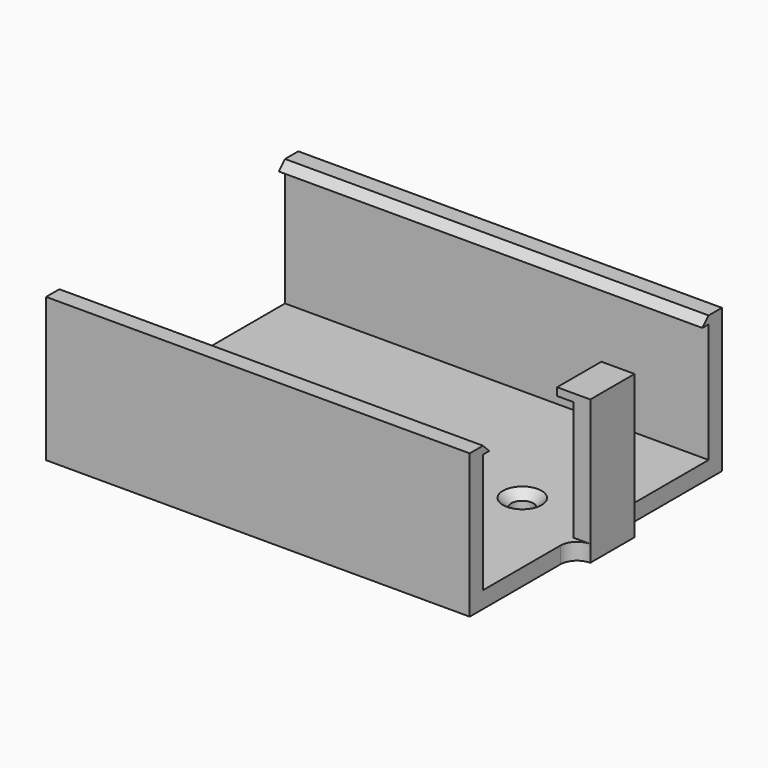
from build123d import *

# Parameters (mm, degrees)
F1_DEPTH        = 38.3
F2_W            = 76.6
F2_H            = 51
F3_DEPTH        = 19.6
F5_DEPTH        = 76.6
F7_DEPTH        = 3
F8_W            = 10
F8_H            = 21.6
F9_DEPTH        = 3
F10_R           = 2.99999
F12_D           = 4
F12_CSINK_D     = 7
F12_CSINK_ANGLE = 90


# Not quite as in the source:
# - a fillet or chamfer is up to 0.001 mm smaller than in the source, because OpenCascade refuses the exact size


with BuildPart() as f1:
    # F0 (on Right) → F1 (new body, symmetric)
    with BuildSketch(Plane.YZ):
        Polygon((-28.5, 13), (-28.5, -13), (-5, -13), (0, -13), (5, -13), (28.5, -13), (28.5, 13), (5, 13), (-5, 13), align=None)
        Polygon((-5, -10), (-25.5, -10), (-25.5, 10), (-5, 10), (5, 10), (25.5, 10), (25.5, -10), (5, -10), align=None, mode=Mode.SUBTRACT)
    extrude(amount=F1_DEPTH, both=True)

    # F2 (on face) → F3 (cut)
    with BuildSketch(Plane.XY.offset(13)):
        Rectangle(F2_W, F2_H)
    extrude(amount=-F3_DEPTH, mode=Mode.SUBTRACT)

    # F4 (on face) → F5 (join)
    with BuildSketch(Plane.YZ.offset(38.3)):
        Polygon((24.0857864376, 11.5857864376), (25.5, 11.5857864376), (25.5, 13), align=None)
        Polygon((-24.0857864376, 11.5857864376), (-25.5, 13), (-25.5, 11.5857864376), align=None)
    extrude(amount=-F5_DEPTH)

    # F6 (on face) → F7 (join, symmetric)
    with BuildSketch(Plane.YZ.offset(38.3)):
        Polygon((-5, -13), (0, -13), (5, -13), (5, 13), (-5, 13), align=None)
    extrude(amount=F7_DEPTH, both=True)

    # F8 (on face) → F9 (cut)
    with BuildSketch(Plane(origin=(35.3, 0, 0), x_dir=(0, -1, 0), z_dir=(-1, 0, 0))):
        with Locations((0, 0.8)):
            Rectangle(F8_W, F8_H)
    extrude(amount=-F9_DEPTH, mode=Mode.SUBTRACT)

    # F10 (radius 3 in the source; OpenCascade refuses exactly that, so slightly less here)
    f10_edges = [f1.edges().sort_by_distance(p)[0] for p in [
        (38.3, -5, -11.5),
        (38.3, 5, -11.5),
    ]]
    fillet(f10_edges, radius=F10_R)

    # F12 (through all)
    with Locations(Plane.XY.offset(-10)):
        with Locations((-25, 0), (25, 0)):
            CounterSinkHole(F12_D / 2, F12_CSINK_D / 2, counter_sink_angle=F12_CSINK_ANGLE)


solid = f1.part
